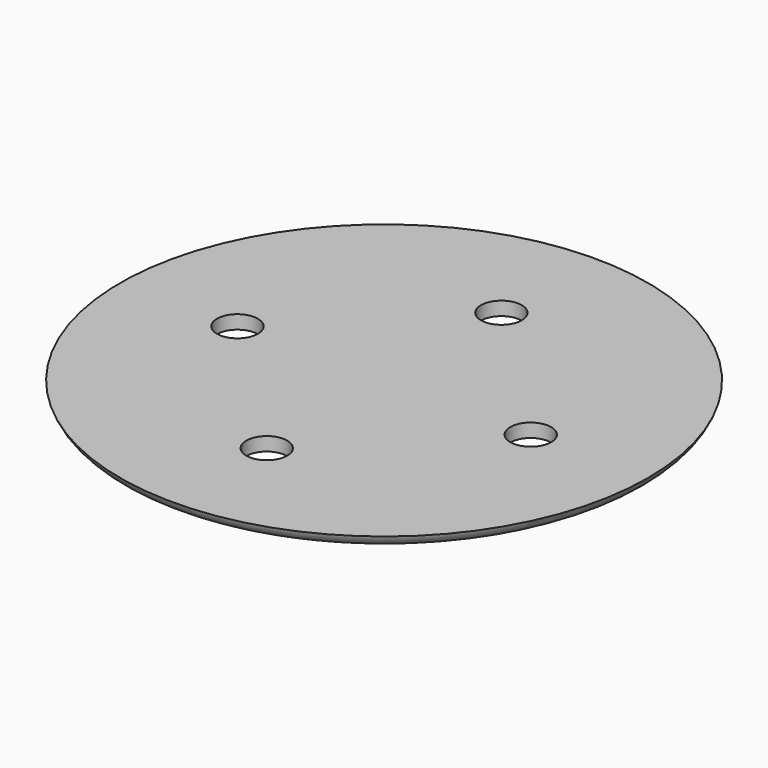
from build123d import *

# Parameters (mm, degrees)
F0_R     = 38.7
F0_R_2   = 3
F1_DEPTH = 2


# Not quite as in the source:
# - a fillet or chamfer that OpenCascade refuses, or shapes differently, is made with other operations: its cross-section is extruded or revolved along the edge and cut away or added


with BuildPart() as f1:
    # F0 (on Top) → F1 (new body)
    with BuildSketch(Plane.XY):
        Circle(F0_R)
        with Locations((0, -21.5)):
            Circle(F0_R_2, mode=Mode.SUBTRACT)
        with Locations((-21.5, 0)):
            Circle(F0_R_2, mode=Mode.SUBTRACT)
        with Locations((21.5, 0)):
            Circle(F0_R_2, mode=Mode.SUBTRACT)
        with Locations((0, 21.5)):
            Circle(F0_R_2, mode=Mode.SUBTRACT)
    extrude(amount=F1_DEPTH)

    # F2: fillet of radius 3 on 1 edges, made by hand

    # F2_s1 → F2_t2 (revolve, cut)
    with BuildSketch(Plane.XZ):
        with BuildLine():
            ThreePointArc((38.7, 2), (37.6036236828, 0.5505102572), (35.8715728753, 0))
            Line((35.8715728753, 0), (38.7, 0))
            Line((38.7, 0), (38.7, 2))
        make_face()
    revolve(axis=Axis((0, 0, 0), (0, 0, 1)), mode=Mode.SUBTRACT)


solid = f1.part
